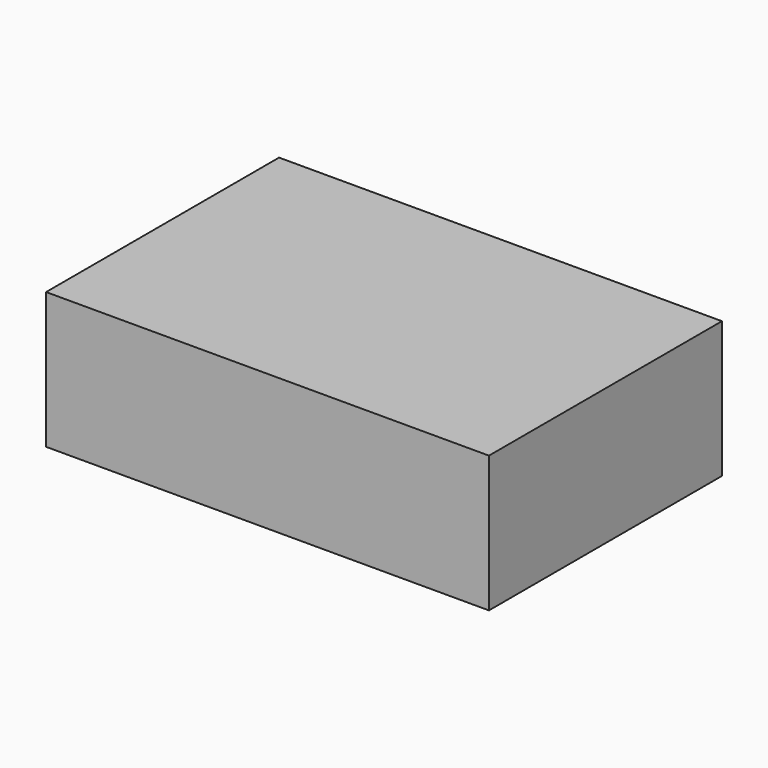
from build123d import *

# Parameters (mm, degrees)
F0_W     = 82.5544893742
F0_H     = 54.2824026197
F1_DEPTH = 25.4


# Not quite as in the source:
# - the program builds the solid bodies; features that only make, move or delete a surface that nothing else refers to are left out


with BuildPart() as f1:
    # F0 (on Top) → F1 (new body)
    with BuildSketch(Plane.XY):
        with Locations((9.4240307808, -2.1675275639)):
            Rectangle(F0_W, F0_H)
    extrude(amount=F1_DEPTH)


solid = f1.part
